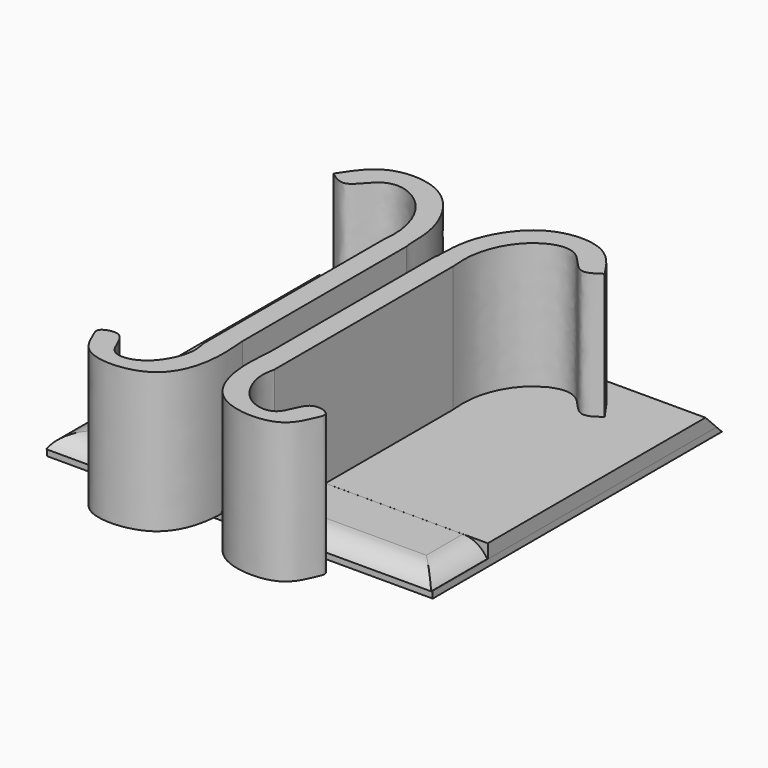
from build123d import *

# Parameters (mm, degrees)
F1_DEPTH     = 25.4
F4_W         = 69.7987195548
F4_H         = 12.7
F5_DEPTH     = 2.54
F6_T1_DEPTH  = 91.7957648109
F7_T1_DEPTH  = 30.2976362049
F8_T1_DEPTH  = 30.2976362049
F9_W         = 69.9951983988
F9_H         = 56.9309936836
F10_DEPTH    = 2.54
F11_W        = 69.9400268495
F11_H        = 66.7930708891
F12_DEPTH    = 1.27
F13_T1_DEPTH = 109.1876471354
F14_T1_DEPTH = 83.0041764284


# Not quite as in the source:
# - a fillet or chamfer that OpenCascade refuses, or shapes differently, is made with other operations: its cross-section is extruded or revolved along the edge and cut away or added


with BuildPart() as f1:
    # F0 (on Top) → F1 (new body)
    with BuildSketch(Plane.XY):
        with BuildLine():
            add(Edge.make_bspline(
                [(-25.3892242908, 29.1687585413), (-23.9101314013, 31.4486866753), (-20.7881663251, 36.2609983704), (-9.1463899399, 35.7254461506), (-3.2777537007, 25.5380991998), (-3.5742881653, 19.1688234613), (-3.3841941276, 18.4209676857), (-3.3333937172, 18.2211119682)],
                knots=[0, 0, 0, 0, 0.2228253831, 0.4703241216, 0.7365451299, 0.9295947644, 1, 1, 1, 1], degree=3))
            add(Edge.make_bspline(
                [(-7.2106076404, 17.4659974873), (-7.0960839892, 18.9182648401), (-6.8460158254, 22.0893637897), (-8.9625216947, 28.2814027293), (-13.8811242457, 32.206810347), (-18.8078127809, 32.0506891323), (-21.8172896516, 26.6531796951), (-24.2679202869, 28.3790664228), (-25.3892242908, 29.1687585413)],
                knots=[0, 0, 0, 0, 0.1607433504, 0.3509912061, 0.535196632, 0.6915441839, 0.8588637812, 1, 1, 1, 1], degree=3))
            Line((-7.2106076404, 17.4659974873), (-7.2106076404, -22.9408182204))
            add(Edge.make_bspline(
                [(-3.3333937172, -18.9407765865), (-3.1142473062, -21.5798728563), (-2.6671599952, -26.9639740582), (-6.2224863176, -36.1495419675), (-18.7613568768, -36.6643913981), (-20.7940116277, -31.023866226), (-22.1012345625, -28.6408761942), (-17.1327960007, -27.1867369593), (-16.4969316925, -34.1062525933), (-9.5670200889, -33.0225376657), (-6.484504483, -26.5775936324), (-6.9952909898, -24.0192576859), (-7.2106076404, -22.9408182204)],
                knots=[0, 0, 0, 0, 0.1210737943, 0.2470063593, 0.3836118826, 0.4813711357, 0.5410941326, 0.6166345084, 0.7128727302, 0.8092971236, 0.919611219, 1, 1, 1, 1], degree=3))
            Line((-3.3333937172, -18.9407765865), (-3.3333937172, 18.2211119682))
        make_face()
    extrude(amount=F1_DEPTH)


with BuildPart() as f3_1:
    # F3: instance of F1
    add(f1.part.mirror(Plane(origin=(-0.7933937172, -0.3598323092, 12.7), x_dir=(0, 1, 0), z_dir=(1, 0, 0))))


with BuildPart() as f5:
    # F4 (on Top) → F5 (new body)
    with BuildSketch(Plane.XY):
        with Locations((0.0479891896, -17.7361853421)):
            Rectangle(F4_W, F4_H)
    extrude(amount=F5_DEPTH)

    # F6: fillet of radius 5.08 on 1 edges, made by hand

    # F6_s2 → F6_t1 (cut)
    with BuildSketch(Plane.YZ.offset(-45.8498932158)):
        with BuildLine():
            ThreePointArc((-24.0861853421, 0), (-22.2267762908, 1.8594090512), (-19.6867762908, 2.54))
            Line((-19.6867762908, 2.54), (-24.0861853421, 2.54))
            Line((-24.0861853421, 2.54), (-24.0861853421, 0))
        make_face()
    extrude(amount=F6_T1_DEPTH, mode=Mode.SUBTRACT)

    # F7: fillet of radius 5.08 on 1 edges, made by hand

    # F7_s2 → F7_t1 (cut)
    with BuildSketch(Plane.XZ.offset(0.387662714)):
        with BuildLine():
            ThreePointArc((-34.8513705878, 0), (-32.9919615365, 1.8594090512), (-30.4519615365, 2.54))
            Line((-30.4519615365, 2.54), (-34.8513705878, 2.54))
            Line((-34.8513705878, 2.54), (-34.8513705878, 0))
        make_face()
    extrude(amount=F7_T1_DEPTH, mode=Mode.SUBTRACT)

    # F8: fillet of radius 5.08 on 1 edges, made by hand

    # F8_s2 → F8_t1 (cut)
    with BuildSketch(Plane.XZ.offset(0.387662714)):
        with BuildLine():
            ThreePointArc((30.5479399158, 2.54), (33.0879399158, 1.8594090512), (34.947348967, 0))
            Line((34.947348967, 0), (34.947348967, 2.54))
            Line((34.947348967, 2.54), (30.5479399158, 2.54))
        make_face()
    extrude(amount=F8_T1_DEPTH, mode=Mode.SUBTRACT)


with BuildPart() as f10:
    # F9 (on Top) → F10 (new body)
    with BuildSketch(Plane.XY):
        with Locations((0.0482033938, 17.0871145092)):
            Rectangle(F9_W, F9_H)
    extrude(amount=F10_DEPTH)

    # F13: chamfer of 7.62 on 1 edges, made by hand

    # F13_s2 → F13_t1 (cut)
    with BuildSketch(Plane.YZ.offset(-54.5456201739)):
        Polygon((45.552611351, -5.08), (37.932611351, 2.54), (45.552611351, 2.54), align=None)
    extrude(amount=F13_T1_DEPTH, mode=Mode.SUBTRACT)


with BuildPart() as f12:
    # F11 (on face) → F12 (new body)
    with BuildSketch(Plane(origin=(0, 0, 0), x_dir=(1, 0, 0), z_dir=(0, 0, -1))):
        with Locations((0.0206176192, -9.6160759065)):
            Rectangle(F11_W, F11_H)
    extrude(amount=F12_DEPTH)

    # F14: chamfer of 2.54 on 1 edges, made by hand

    # F14_s2 → F14_t1 (cut)
    with BuildSketch(Plane.YZ.offset(-41.481470595)):
        Polygon((43.012611351, -2.54), (40.472611351, 0), (43.012611351, 0), align=None)
    extrude(amount=F14_T1_DEPTH, mode=Mode.SUBTRACT)


solid = Compound([f1.part, f3_1.part, f5.part, f10.part, f12.part])
